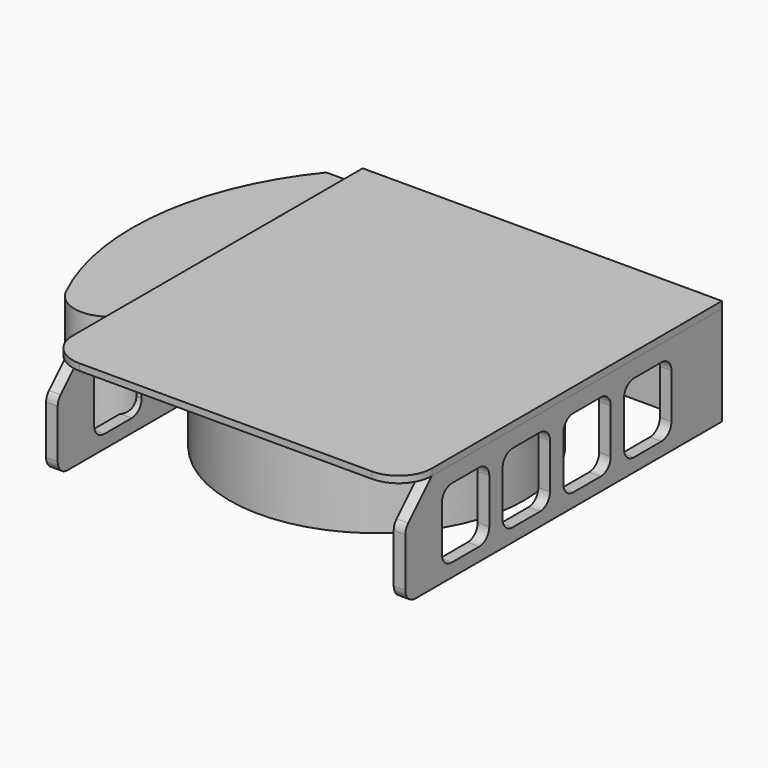
from build123d import *

# Parameters (mm, degrees)
F2_R          = 177.5
F3_DEPTH      = 90
F4_W          = 117
F4_H          = 40
F5_DEPTH      = 5
F5_DEPTH_BACK = 90
F7_DEPTH      = 4.5
F10_W         = 202.5
F10_H         = 120
F11_DEPTH     = 16
F14_W         = 71.5
F14_H         = 84
F15_DEPTH     = 14
F17_R         = 15
F22_DEPTH     = 8
F24_DEPTH     = 120


# Not quite as in the source:
# - a feature names something its author has since deleted; it is built from what else it names


with BuildPart() as f3:
    # F2 (on plane+point) → F3 (new body)
    with BuildSketch(Plane.XY.offset(5)):
        Circle(F2_R)
    extrude(amount=F3_DEPTH)


with BuildPart() as f5:
    # F4 (on plane+point) → F5 (new body, two sides)
    with BuildSketch(Plane.XY.offset(5)) as f5_sk:
        with Locations((0, 207.5)):
            Rectangle(F4_W, F4_H)
    extrude(amount=-F5_DEPTH)
    extrude(f5_sk.sketch, amount=F5_DEPTH_BACK)

    # F6 (on Top) → F7 (join)
    with BuildSketch(Plane.XY):
        with BuildLine():
            Line((59, 232.5), (-59, 232.5))
            ThreePointArc((-59, 232.5), (-63.9497474683, 230.4497474683), (-66, 225.5))
            Line((-66, 225.5), (-66, 94.5))
            ThreePointArc((-66, 94.5), (-63.9497474683, 89.5502525317), (-59, 87.5))
            Line((-59, 87.5), (59, 87.5))
            ThreePointArc((59, 87.5), (63.9497474683, 89.5502525317), (66, 94.5))
            Line((66, 94.5), (66, 225.5))
            ThreePointArc((66, 225.5), (63.9497474683, 230.4497474683), (59, 232.5))
        make_face()
    extrude(amount=F7_DEPTH)


with BuildPart() as f11:
    # F10 (on plane+point) → F11 (new body)
    with BuildSketch(Plane.XZ.offset(-233.5)):
        with Locations((-101.25, 60)):
            Rectangle(F10_W, F10_H)
    extrude(amount=-F11_DEPTH)


with BuildPart() as f15:
    # F14 (on face) → F15 (new body)
    with BuildSketch(Plane(origin=(-202.5, 0, 0), x_dir=(0, -1, 0), z_dir=(-1, 0, 0))):
        Polygon((187.5, 120), (-249.5, 120), (-249.5, 0), (227.5, 0), (227.5, 80), align=None)
        with Locations((-137.75, 58)):
            Rectangle(F14_W, F14_H, mode=Mode.SUBTRACT)
        with Locations((-46.25, 58)):
            Rectangle(F14_W, F14_H, mode=Mode.SUBTRACT)
        with Locations((45.25, 58)):
            Rectangle(F14_W, F14_H, mode=Mode.SUBTRACT)
        with Locations((136.75, 58)):
            Rectangle(F14_W, F14_H, mode=Mode.SUBTRACT)
    extrude(amount=F15_DEPTH)

    # F17
    f17_edges = [f15.edges().sort_by_distance(p)[0] for p in [
        (-209.5, 82, 100),
        (-209.5, 173.5, 100),
        (-209.5, -227.5, 0),
        (-209.5, -227.5, 80),
        (-209.5, 173.5, 16),
        (-209.5, 10.5, 16),
        (-209.5, 102, 16),
        (-209.5, 102, 100),
        (-209.5, -101, 16),
        (-209.5, -172.5, 16),
        (-209.5, -172.5, 100),
        (-209.5, -101, 100),
        (-209.5, -9.5, 16),
        (-209.5, -9.5, 100),
        (-209.5, -81, 16),
        (-209.5, -81, 100),
        (-209.5, 10.5, 100),
        (-209.5, 82, 16),
    ]]
    fillet(f17_edges, radius=F17_R)


with BuildPart() as f18_1:
    # F18: instance of F11
    add(f11.part.mirror(Plane.YZ))


with BuildPart() as f19_1:
    # F19: instance of F15
    add(f15.part.mirror(Plane.YZ))


with BuildPart() as f22:
    # F21 (on plane+point) → F22 (new body)
    with BuildSketch(Plane.XY.offset(120)):
        with BuildLine():
            Line((216.5, -187.5), (216.5, 249.5))
            Line((216.5, 249.5), (-216.5, 249.5))
            Line((-216.5, 249.5), (-216.5, -187.5))
            ThreePointArc((-216.5, -187.5), (-204.7842712475, -215.7842712475), (-176.5, -227.5))
            Line((-176.5, -227.5), (176.5, -227.5))
            ThreePointArc((176.5, -227.5), (204.7842712475, -215.7842712475), (216.5, -187.5))
        make_face()
    extrude(amount=F22_DEPTH)


with BuildPart() as f11_1:
    add(f11.part)

    # F23: union F18_1
    add(f18_1.part)


with BuildPart() as f24:
    # F12 (on face) → F24 (new body, through all)
    with BuildSketch(Plane(origin=(0, 0, 0), x_dir=(1, 0, 0), z_dir=(0, 0, -1))):
        with BuildLine():
            ThreePointArc((-287.2044828435, 109.2236505243), (-317.5294909897, -67.9642915883), (-247.435966397, -233.5))
            Line((-247.435966397, -233.5), (-202.5, -233.5))
            Line((-202.5, -233.5), (-71, -233.5))
            Line((-71, -233.5), (-71, -203.5))
            ThreePointArc((-71, -203.5), (-78.2339182284, -180.556942546), (-97.319194267, -165.9122951686))
            ThreePointArc((-97.319194267, -165.9122951686), (-177.2164384695, -104.6049834268), (-207.5, -8.5577970797))
            Line((-207.5, -8.5577970797), (-207.5, 90.791272666))
            ThreePointArc((-207.5, 90.791272666), (-240.0241445264, 131.6952979534), (-287.2044828435, 109.2236505243))
        make_face()
    extrude(amount=-F24_DEPTH)


solid = Compound([f3.part, f5.part, f15.part, f19_1.part, f22.part, f11_1.part, f24.part])
